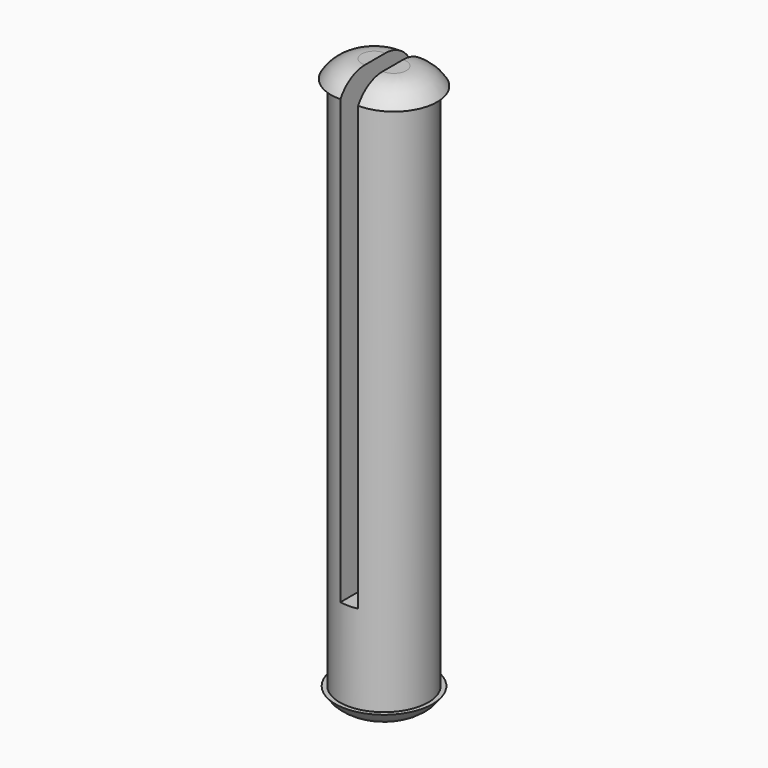
from build123d import *

# Parameters (mm, degrees)
F0_R        = 6.35
F1_DEPTH    = 76.2
F3_DEPTH    = 63.5
F5_DEPTH    = 2.54
F6_T4_ANGLE = 359.64
F6_T9_ANGLE = 359.64
F7_R        = 6.985
F7_R_2      = 6.35
F8_DEPTH    = 2.54


# Not quite as in the source:
# - a fillet or chamfer that OpenCascade refuses, or shapes differently, is made with other operations: its cross-section is extruded or revolved along the edge and cut away or added


with BuildPart() as f1:
    # F0 (on Top) → F1 (new body)
    with BuildSketch(Plane.XY):
        Circle(F0_R)
    extrude(amount=F1_DEPTH)

    # F2 (on face) → F3 (cut)
    with BuildSketch(Plane.XY.offset(76.2)):
        with BuildLine():
            Line((1.27, -6.2217039467), (1.27, 6.2217039467))
            ThreePointArc((1.27, 6.2217039467), (0, 6.35), (-1.27, 6.2217039467))
            Line((-1.27, 6.2217039467), (-1.27, -6.2217039467))
            ThreePointArc((-1.27, -6.2217039467), (0, -6.35), (1.27, -6.2217039467))
        make_face()
    extrude(amount=-F3_DEPTH, mode=Mode.SUBTRACT)

    # F4 (on face) → F5 (join)
    with BuildSketch(Plane.XY.offset(76.2)):
        with BuildLine():
            ThreePointArc((-1.27, -6.2217039467), (-6.35, 0), (-1.27, 6.2217039467))
            ThreePointArc((-1.27, 6.2217039467), (-7.62, 0), (-1.27, -6.2217039467))
        make_face()
        with BuildLine():
            Line((-1.27, -6.2217039467), (-1.27, 6.2217039467))
            ThreePointArc((-1.27, 6.2217039467), (-6.35, 0), (-1.27, -6.2217039467))
        make_face()
        with BuildLine():
            ThreePointArc((1.27, -6.2217039467), (7.62, 0), (1.27, 6.2217039467))
            Line((1.27, 6.2217039467), (1.27, -6.2217039467))
        make_face()
    extrude(amount=F5_DEPTH)

    # F6: fillet of radius 5.08 on 2 edges, made by hand


with BuildPart() as f6_tool2:
    # F6_s3 → F6_t4 (revolve)
    with BuildSketch(Plane(origin=(-1.37878e-05, 0.0043887761, 0), x_dir=(0, 0, 1), z_dir=(0.0031415875, -0.9999950652, 0))):
        with BuildLine():
            ThreePointArc((76.2, -4.8260068939), (78.0594090512, -2.9665978427), (78.74, -0.4265978427))
            Line((78.74, -0.4265978427), (78.74, -4.8260068939))
            Line((78.74, -4.8260068939), (76.2, -4.8260068939))
        make_face()
    revolve(axis=Axis((-1.397, 0, 78.74), (0, 0, 1)), revolution_arc=F6_T4_ANGLE)

    split(bisect_by=Plane.YZ.offset(-1.27), keep=Keep.BOTTOM)


with BuildPart() as f1_1:
    add(f1.part)

    # F6_t1: cut F6_tool2
    add(f6_tool2.part, mode=Mode.SUBTRACT)


with BuildPart() as f6_tool7:
    # F6_s8 → F6_t9 (revolve)
    with BuildSketch(Plane(origin=(1.37878e-05, -0.0043887761, 0), x_dir=(0, 0, 1), z_dir=(-0.0031415875, 0.9999950652, 0))):
        with BuildLine():
            ThreePointArc((76.2, -4.8260068939), (78.0594090512, -2.9665978427), (78.74, -0.4265978427))
            Line((78.74, -0.4265978427), (78.74, -4.8260068939))
            Line((78.74, -4.8260068939), (76.2, -4.8260068939))
        make_face()
    revolve(axis=Axis((1.397, 0, 78.74), (0, 0, 1)), revolution_arc=F6_T9_ANGLE)

    split(bisect_by=Plane.YZ.offset(-1.27), keep=Keep.TOP)


with BuildPart() as f1_2:
    add(f1_1.part)

    # F6_t6: cut F6_tool7
    add(f6_tool7.part, mode=Mode.SUBTRACT)

    # F7 (on face) → F8 (join)
    with BuildSketch(Plane(origin=(0, 0, 0), x_dir=(1, 0, 0), z_dir=(0, 0, -1))):
        Circle(F7_R)
        Circle(F7_R_2, mode=Mode.SUBTRACT)
        Circle(F7_R_2)
    extrude(amount=F8_DEPTH)

    # F9: fillet of radius 5.08 on 1 edges, made by hand

    # F9_s1 → F9_t2 (revolve, cut)
    with BuildSketch(Plane.XZ):
        with BuildLine():
            ThreePointArc((6.985, 0), (5.1255909488, -1.8594090512), (2.5855909488, -2.54))
            Line((2.5855909488, -2.54), (2.5855909488, -2.6416))
            Line((2.5855909488, -2.6416), (6.985, -2.6416))
            Line((6.985, -2.6416), (7.0866, -2.54))
            ThreePointArc((7.0866, -2.54), (7.0866, -1.27), (7.072988181, -0.0508))
            Line((7.072988181, -0.0508), (6.985, 0))
        make_face()
    revolve(axis=Axis((0, 0, -2.54), (0, 0, -1)), mode=Mode.SUBTRACT)


solid = f1_2.part
